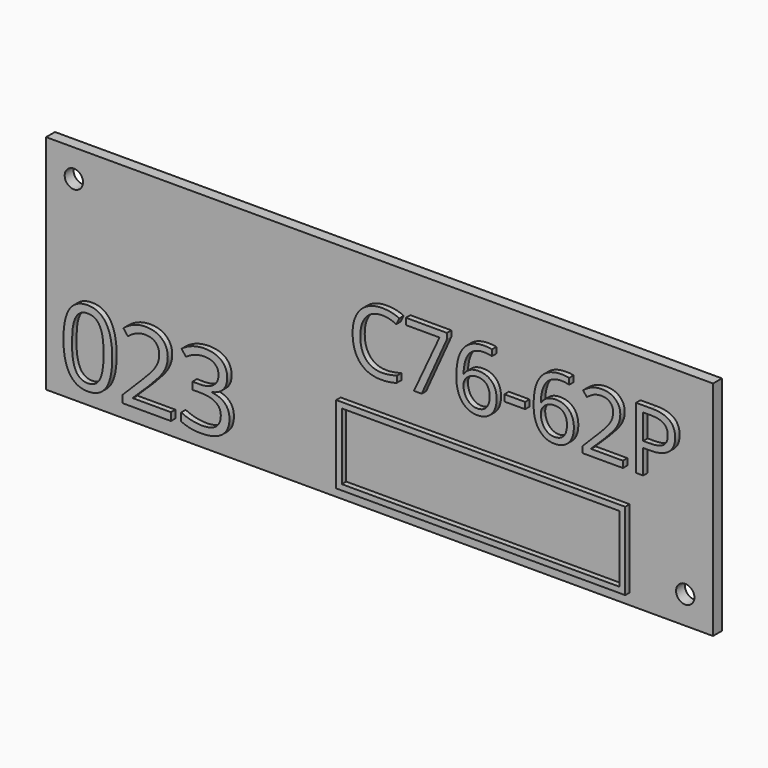
from build123d import *

# Parameters (mm, degrees)
F0_W         = 120
F0_H         = 40
F1_DEPTH     = 2
F3_D         = 3.3
F4_TEXT_SIZE = 15.5635715154
F5_DEPTH     = 1
F6_TEXT_SIZE = 18.5894526641
F7_DEPTH     = 1
F8_W         = 52
F8_H         = 14
F8_W_2       = 49.99999962
F8_H_2       = 11.99999962
F9_DEPTH     = 1


# Not quite as in the source:
# - Text() gives the source's letters only with a copy of the font that has no kerning and outlines rounded to 1/6400 em; it was checked with that copy


with BuildPart() as f1:
    # F0 (on Front) → F1 (new body)
    with BuildSketch(Plane.XZ):
        Rectangle(F0_W, F0_H)
    extrude(amount=F1_DEPTH)

    # F3 (through all)
    with Locations(Plane.XZ.offset(2)):
        with Locations((-55, 15), (55, -15)):
            Hole(F3_D / 2)

    # F4 (on face) → F5 (join)
    with BuildSketch(Plane.XZ.offset(2)):
        with Locations((-5, 2)):
            Text('C76-62P', F4_TEXT_SIZE, font='Open Sans', text_align=(TextAlign.LEFT, TextAlign.BOTTOM))
    extrude(amount=F5_DEPTH)

    # F6 (on face) → F7 (join)
    with BuildSketch(Plane.XZ.offset(2)):
        with Locations((-57, -17)):
            Text('023', F6_TEXT_SIZE, font='Open Sans', text_align=(TextAlign.LEFT, TextAlign.BOTTOM))
    extrude(amount=F7_DEPTH)

    # F8 (on face) → F9 (join)
    with BuildSketch(Plane.XZ.offset(2)):
        with Locations((19, -11)):
            Rectangle(F8_W, F8_H)
        with Locations((19, -11)):
            Rectangle(F8_W_2, F8_H_2, mode=Mode.SUBTRACT)
    extrude(amount=F9_DEPTH)


solid = f1.part
